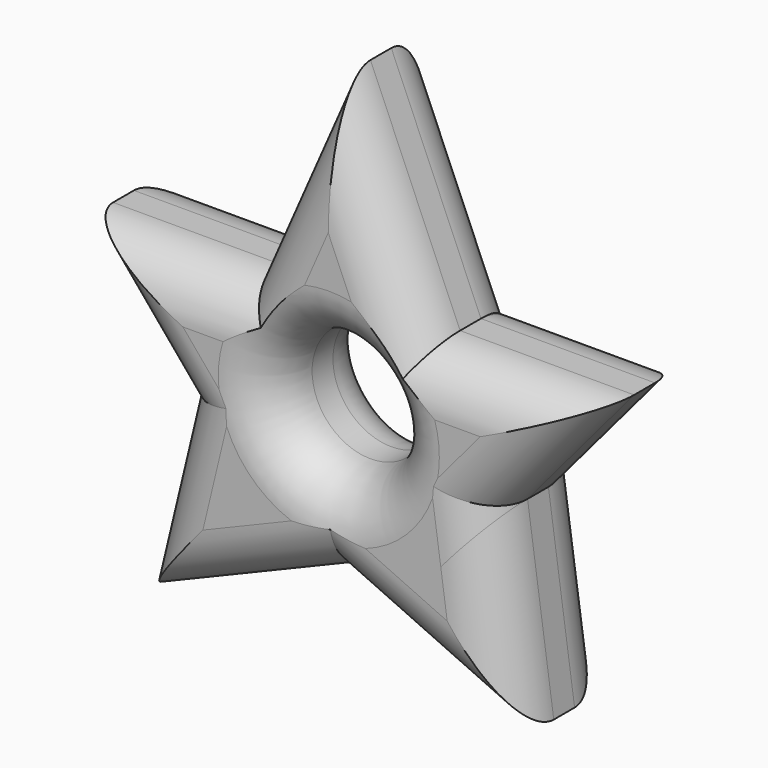
from build123d import *

# Parameters (mm, degrees)
F0_R          = 5.6926313443
F1_DEPTH      = 12.7
F2_T4_DEPTH   = 43.6889551243
F2_T9_DEPTH   = 41.5057154141
F2_T14_DEPTH  = 42.3716066055
F2_T19_DEPTH  = 47.5765515209
F2_T24_DEPTH  = 47.6597095959
F2_T29_DEPTH  = 41.5552379071
F2_T34_DEPTH  = 40.9570702629
F2_T39_DEPTH  = 44.4053400631
F2_T44_DEPTH  = 46.5690535596
F2_T49_DEPTH  = 45.0341334131
F2_T56_DEPTH  = 43.6889551243
F2_T61_DEPTH  = 41.5057154141
F2_T66_DEPTH  = 42.3716066055
F2_T71_DEPTH  = 47.5765515209
F2_T76_DEPTH  = 47.6597095959
F2_T81_DEPTH  = 41.5552379071
F2_T86_DEPTH  = 40.9570702629
F2_T91_DEPTH  = 44.4053400631
F2_T96_DEPTH  = 46.5690535596
F2_T101_DEPTH = 45.0341334131
F2_T109_DEPTH = 43.6889551243
F2_T113_DEPTH = 41.5057154141
F2_T120_DEPTH = 42.3716066055
F2_T124_DEPTH = 47.5765515209
F2_T131_DEPTH = 47.6597095959
F2_T135_DEPTH = 41.5552379071
F2_T142_DEPTH = 40.9570702629
F2_T146_DEPTH = 44.4053400631
F2_T153_DEPTH = 46.5690535596
F2_T157_DEPTH = 45.0341334131
F2_T164_DEPTH = 43.6889551243
F2_T168_DEPTH = 41.5057154141
F2_T175_DEPTH = 42.3716066055
F2_T179_DEPTH = 47.5765515209
F2_T186_DEPTH = 47.6597095959
F2_T190_DEPTH = 41.5552379071
F2_T197_DEPTH = 40.9570702629
F2_T201_DEPTH = 44.4053400631
F2_T208_DEPTH = 46.5690535596
F2_T212_DEPTH = 45.0341334131


# Not quite as in the source:
# - a fillet or chamfer that OpenCascade refuses, or shapes differently, is made with other operations: its cross-section is extruded or revolved along the edge and cut away or added


with BuildPart() as f1:
    # F0 (on Front) → F1 (new body)
    with BuildSketch(Plane.XZ):
        Polygon((25.7036406547, 22.2720243037), (8.7320340492, 22.2720243037), (0, 42.6570928276), (-8.9411214382, 22.2720243037), (-25.0963593453, 22.2720243037), (-15.1141012942, 10.3398426354), (-19.5402633399, -8.1429071724), (0, 0), (17.8659524701, -8.1429071724), (15.3123920323, 9.9669025623), align=None)
        with Locations((0, 14.1210428621)):
            Circle(F0_R, mode=Mode.SUBTRACT)
    extrude(amount=F1_DEPTH)

    # F2: fillet of radius 5.08 on 22 edges, made by hand


with BuildPart() as f2_tool2:
    # F2_s3 → F2_t4 (new body)
    with BuildSketch(Plane(origin=(3.2473042237, 0, -23.0298295556), x_dir=(0, 1, 0), z_dir=(-0.1396230906, 0, 0.9902047226))):
        with BuildLine():
            ThreePointArc((-7.62, -16.5540126433), (-11.2121024484, -15.0661150917), (-12.7, -11.4740126433))
            Line((-12.7, -11.4740126433), (-12.7, -16.5540126433))
            Line((-12.7, -16.5540126433), (-7.62, -16.5540126433))
        make_face()
    extrude(amount=F2_T4_DEPTH)

    split(bisect_by=Plane(origin=(4.0252181101, 0, -3.3991571169), x_dir=(0, 1, 0), z_dir=(0.7640220521, 0, -0.64519013)), keep=Keep.TOP)


with BuildPart() as f1_1:
    add(f1.part)

    # F2_t1: cut F2_tool2
    add(f2_tool2.part, mode=Mode.SUBTRACT)


with BuildPart() as f2_tool7:
    # F2_s8 → F2_t9 (new body)
    with BuildSketch(Plane(origin=(3.0932592707, 0, 3.6629796175), x_dir=(0, 1, 0), z_dir=(0.64519013, 0, 0.7640220521))):
        with BuildLine():
            ThreePointArc((-7.62, -5.2684580229), (-11.2121024484, -3.7805604713), (-12.7, -0.1884580229))
            Line((-12.7, -0.1884580229), (-12.7, -5.2684580229))
            Line((-12.7, -5.2684580229), (-7.62, -5.2684580229))
        make_face()
    extrude(amount=F2_T9_DEPTH)

    split(bisect_by=Plane(origin=(16.3918614967, 0, 2.3113224066), x_dir=(0, 1, 0), z_dir=(0.9902047226, 0, 0.1396230906)), keep=Keep.TOP)


with BuildPart() as f1_2:
    add(f1_1.part)

    # F2_t6: cut F2_tool7
    add(f2_tool7.part, mode=Mode.SUBTRACT)


with BuildPart() as f2_tool12:
    # F2_s13 → F2_t14 (new body)
    with BuildSketch(Plane.YZ.offset(38.4036406547)):
        with BuildLine():
            ThreePointArc((-7.62, 22.2720243037), (-11.2121024484, 20.7841267521), (-12.7, 17.1920243037))
            Line((-12.7, 17.1920243037), (-12.7, 22.2720243037))
            Line((-12.7, 22.2720243037), (-7.62, 22.2720243037))
        make_face()
    extrude(amount=-F2_T14_DEPTH)

    split(bisect_by=Plane(origin=(15.4394143514, 0, 6.6135412622), x_dir=(0, 1, 0), z_dir=(0.9192172419, 0, 0.3937507615)), keep=Keep.TOP)


with BuildPart() as f1_3:
    add(f1_2.part)

    # F2_t11: cut F2_tool12
    add(f2_tool12.part, mode=Mode.SUBTRACT)


with BuildPart() as f2_tool17:
    # F2_s18 → F2_t19 (new body)
    with BuildSketch(Plane(origin=(-1.706745631, 0, 3.9844240694), x_dir=(0, 1, 0), z_dir=(-0.3937507615, 0, 0.9192172419))):
        with BuildLine():
            ThreePointArc((-7.62, -16.7962627849), (-11.2121024484, -15.3083652333), (-12.7, -11.7162627849))
            Line((-12.7, -11.7162627849), (-12.7, -16.7962627849))
            Line((-12.7, -16.7962627849), (-7.62, -16.7962627849))
        make_face()
    extrude(amount=F2_T19_DEPTH)

    split(bisect_by=Plane.XY.offset(22.2720243037), keep=Keep.TOP)


with BuildPart() as f1_4:
    add(f1_3.part)

    # F2_t16: cut F2_tool17
    add(f2_tool17.part, mode=Mode.SUBTRACT)


with BuildPart() as f2_tool22:
    # F2_s23 → F2_t24 (new body)
    with BuildSketch(Plane(origin=(20.7924554538, 0, 47.4051976742), x_dir=(0, 1, 0), z_dir=(-0.40167287, 0, -0.9157832197))):
        with BuildLine():
            ThreePointArc((-7.62, -17.1341969008), (-11.2121024484, -15.6462993492), (-12.7, -12.0541969008))
            Line((-12.7, -12.0541969008), (-12.7, -17.1341969008))
            Line((-12.7, -17.1341969008), (-7.62, -17.1341969008))
        make_face()
    extrude(amount=F2_T24_DEPTH)

    split(bisect_by=Plane.XY.offset(22.2720243037), keep=Keep.TOP)


with BuildPart() as f1_5:
    add(f1_4.part)

    # F2_t21: cut F2_tool22
    add(f2_tool22.part, mode=Mode.SUBTRACT)


with BuildPart() as f2_tool27:
    # F2_s28 → F2_t29 (new body)
    with BuildSketch(Plane.YZ.offset(3.7588785618)):
        with BuildLine():
            ThreePointArc((-7.62, 22.2720243037), (-11.2121024484, 20.7841267521), (-12.7, 17.1920243037))
            Line((-12.7, 17.1920243037), (-12.7, 22.2720243037))
            Line((-12.7, 22.2720243037), (-7.62, 22.2720243037))
        make_face()
    extrude(amount=-F2_T29_DEPTH)

    split(bisect_by=Plane(origin=(-15.6912100052, 0, 6.8823420438), x_dir=(0, 1, 0), z_dir=(-0.9157832197, 0, 0.40167287)), keep=Keep.TOP)


with BuildPart() as f1_6:
    add(f1_5.part)

    # F2_t26: cut F2_tool27
    add(f2_tool27.part, mode=Mode.SUBTRACT)


with BuildPart() as f2_tool32:
    # F2_s33 → F2_t34 (new body)
    with BuildSketch(Plane(origin=(-29.4427441593, 0, 35.1940583308), x_dir=(0, 1, 0), z_dir=(0.6416541085, 0, -0.7669941362))):
        with BuildLine():
            ThreePointArc((-7.62, -4.9578245582), (-11.2121024484, -3.4699270066), (-12.7, 0.1221754418))
            Line((-12.7, 0.1221754418), (-12.7, -4.9578245582))
            Line((-12.7, -4.9578245582), (-7.62, -4.9578245582))
        make_face()
    extrude(amount=F2_T34_DEPTH)

    split(bisect_by=Plane(origin=(-16.6361796063, 0, 3.9839540936), x_dir=(0, 1, 0), z_dir=(-0.9725029779, 0, 0.2328904419)), keep=Keep.TOP)


with BuildPart() as f1_7:
    add(f1_6.part)

    # F2_t31: cut F2_tool32
    add(f2_tool32.part, mode=Mode.SUBTRACT)


with BuildPart() as f2_tool37:
    # F2_s38 → F2_t39 (new body)
    with BuildSketch(Plane(origin=(4.4797869241, 0, 18.7066763614), x_dir=(0, 1, 0), z_dir=(-0.2328904419, 0, -0.9725029779))):
        with BuildLine():
            ThreePointArc((-7.62, -17.1065590378), (-11.2121024484, -15.6186614862), (-12.7, -12.0265590378))
            Line((-12.7, -12.0265590378), (-12.7, -17.1065590378))
            Line((-12.7, -17.1065590378), (-7.62, -17.1065590378))
        make_face()
    extrude(amount=F2_T39_DEPTH)

    split(bisect_by=Plane(origin=(-3.8026223645, 0, -3.1812084972), x_dir=(0, 1, 0), z_dir=(-0.7669941362, 0, -0.6416541085)), keep=Keep.TOP)


with BuildPart() as f1_8:
    add(f1_7.part)

    # F2_t36: cut F2_tool37
    add(f2_tool37.part, mode=Mode.SUBTRACT)


with BuildPart() as f2_tool42:
    # F2_s43 → F2_t44 (new body)
    with BuildSketch(Plane(origin=(-31.2630993995, 0, -13.0281005893), x_dir=(0, 1, 0), z_dir=(0.9230579574, 0, 0.384660899))):
        with BuildLine():
            ThreePointArc((-7.62, 0), (-11.2121024484, 1.4878975516), (-12.7, 5.08))
            Line((-12.7, 5.08), (-12.7, 0))
            Line((-12.7, 0), (-7.62, 0))
        make_face()
    extrude(amount=F2_T44_DEPTH)

    split(bisect_by=Plane(origin=(0, 0, 0), x_dir=(0, 1, 0), z_dir=(-0.4147321912, 0, -0.90994352)), keep=Keep.TOP)


with BuildPart() as f1_9:
    add(f1_8.part)

    # F2_t41: cut F2_tool42
    add(f2_tool42.part, mode=Mode.SUBTRACT)


with BuildPart() as f2_tool47:
    # F2_s48 → F2_t49 (new body)
    with BuildSketch(Plane(origin=(-11.556282704, 0, 5.2670988281), x_dir=(0, 1, 0), z_dir=(0.90994352, 0, -0.4147321912))):
        with BuildLine():
            ThreePointArc((-7.62, 0), (-11.2121024484, 1.4878975516), (-12.7, 5.08))
            Line((-12.7, 5.08), (-12.7, 0))
            Line((-12.7, 0), (-7.62, 0))
        make_face()
    extrude(amount=F2_T49_DEPTH)

    split(bisect_by=Plane(origin=(0, 0, 0), x_dir=(0, 1, 0), z_dir=(0.384660899, 0, -0.9230579574)), keep=Keep.TOP)


with BuildPart() as f1_10:
    add(f1_9.part)

    # F2_t46: cut F2_tool47
    add(f2_tool47.part, mode=Mode.SUBTRACT)

    # F2_s51 → F2_t52 (revolve, cut)
    with BuildSketch(Plane.XY.offset(14.1210428621)):
        with BuildLine():
            ThreePointArc((5.6926313443, -7.62), (7.1805288959, -11.2121024484), (10.7726313443, -12.7))
            Line((10.7726313443, -12.7), (5.6926313443, -12.7))
            Line((5.6926313443, -12.7), (5.6926313443, -7.62))
        make_face()
    revolve(axis=Axis((0, -12.7, 14.1210428621), (0, -1, 0)), mode=Mode.SUBTRACT)


with BuildPart() as f2_tool54:
    # F2_s55 → F2_t56 (new body)
    with BuildSketch(Plane(origin=(3.2473042237, 0, -23.0298295556), x_dir=(0, 1, 0), z_dir=(-0.1396230906, 0, 0.9902047226))):
        with BuildLine():
            ThreePointArc((-5.08, -16.5540126433), (-1.4878975516, -15.0661150917), (0, -11.4740126433))
            Line((0, -11.4740126433), (0, -16.5540126433))
            Line((0, -16.5540126433), (-5.08, -16.5540126433))
        make_face()
    extrude(amount=F2_T56_DEPTH)

    split(bisect_by=Plane(origin=(4.0252181101, 0, -3.3991571169), x_dir=(0, 1, 0), z_dir=(0.7640220521, 0, -0.64519013)), keep=Keep.TOP)


with BuildPart() as f1_11:
    add(f1_10.part)

    # F2_t53: cut F2_tool54
    add(f2_tool54.part, mode=Mode.SUBTRACT)


with BuildPart() as f2_tool59:
    # F2_s60 → F2_t61 (new body)
    with BuildSketch(Plane(origin=(3.0932592707, 0, 3.6629796175), x_dir=(0, 1, 0), z_dir=(0.64519013, 0, 0.7640220521))):
        with BuildLine():
            ThreePointArc((-5.08, -5.2684580229), (-1.4878975516, -3.7805604713), (0, -0.1884580229))
            Line((0, -0.1884580229), (0, -5.2684580229))
            Line((0, -5.2684580229), (-5.08, -5.2684580229))
        make_face()
    extrude(amount=F2_T61_DEPTH)

    split(bisect_by=Plane(origin=(16.3918614967, 0, 2.3113224066), x_dir=(0, 1, 0), z_dir=(0.9902047226, 0, 0.1396230906)), keep=Keep.TOP)


with BuildPart() as f1_12:
    add(f1_11.part)

    # F2_t58: cut F2_tool59
    add(f2_tool59.part, mode=Mode.SUBTRACT)


with BuildPart() as f2_tool64:
    # F2_s65 → F2_t66 (new body)
    with BuildSketch(Plane.YZ.offset(38.4036406547)):
        with BuildLine():
            ThreePointArc((-5.08, 22.2720243037), (-1.4878975516, 20.7841267521), (0, 17.1920243037))
            Line((0, 17.1920243037), (0, 22.2720243037))
            Line((0, 22.2720243037), (-5.08, 22.2720243037))
        make_face()
    extrude(amount=-F2_T66_DEPTH)

    split(bisect_by=Plane(origin=(15.4394143514, 0, 6.6135412622), x_dir=(0, 1, 0), z_dir=(0.9192172419, 0, 0.3937507615)), keep=Keep.TOP)


with BuildPart() as f1_13:
    add(f1_12.part)

    # F2_t63: cut F2_tool64
    add(f2_tool64.part, mode=Mode.SUBTRACT)


with BuildPart() as f2_tool69:
    # F2_s70 → F2_t71 (new body)
    with BuildSketch(Plane(origin=(-1.706745631, 0, 3.9844240694), x_dir=(0, 1, 0), z_dir=(-0.3937507615, 0, 0.9192172419))):
        with BuildLine():
            ThreePointArc((-5.08, -16.7962627849), (-1.4878975516, -15.3083652333), (0, -11.7162627849))
            Line((0, -11.7162627849), (0, -16.7962627849))
            Line((0, -16.7962627849), (-5.08, -16.7962627849))
        make_face()
    extrude(amount=F2_T71_DEPTH)

    split(bisect_by=Plane.XY.offset(22.2720243037), keep=Keep.TOP)


with BuildPart() as f1_14:
    add(f1_13.part)

    # F2_t68: cut F2_tool69
    add(f2_tool69.part, mode=Mode.SUBTRACT)


with BuildPart() as f2_tool74:
    # F2_s75 → F2_t76 (new body)
    with BuildSketch(Plane(origin=(20.7924554538, 0, 47.4051976742), x_dir=(0, 1, 0), z_dir=(-0.40167287, 0, -0.9157832197))):
        with BuildLine():
            ThreePointArc((-5.08, -17.1341969008), (-1.4878975516, -15.6462993492), (0, -12.0541969008))
            Line((0, -12.0541969008), (0, -17.1341969008))
            Line((0, -17.1341969008), (-5.08, -17.1341969008))
        make_face()
    extrude(amount=F2_T76_DEPTH)

    split(bisect_by=Plane.XY.offset(22.2720243037), keep=Keep.TOP)


with BuildPart() as f1_15:
    add(f1_14.part)

    # F2_t73: cut F2_tool74
    add(f2_tool74.part, mode=Mode.SUBTRACT)


with BuildPart() as f2_tool79:
    # F2_s80 → F2_t81 (new body)
    with BuildSketch(Plane.YZ.offset(3.7588785618)):
        with BuildLine():
            ThreePointArc((-5.08, 22.2720243037), (-1.4878975516, 20.7841267521), (0, 17.1920243037))
            Line((0, 17.1920243037), (0, 22.2720243037))
            Line((0, 22.2720243037), (-5.08, 22.2720243037))
        make_face()
    extrude(amount=-F2_T81_DEPTH)

    split(bisect_by=Plane(origin=(-15.6912100052, 0, 6.8823420438), x_dir=(0, 1, 0), z_dir=(-0.9157832197, 0, 0.40167287)), keep=Keep.TOP)


with BuildPart() as f1_16:
    add(f1_15.part)

    # F2_t78: cut F2_tool79
    add(f2_tool79.part, mode=Mode.SUBTRACT)


with BuildPart() as f2_tool84:
    # F2_s85 → F2_t86 (new body)
    with BuildSketch(Plane(origin=(-29.4427441593, 0, 35.1940583308), x_dir=(0, 1, 0), z_dir=(0.6416541085, 0, -0.7669941362))):
        with BuildLine():
            ThreePointArc((-5.08, -4.9578245582), (-1.4878975516, -3.4699270066), (0, 0.1221754418))
            Line((0, 0.1221754418), (0, -4.9578245582))
            Line((0, -4.9578245582), (-5.08, -4.9578245582))
        make_face()
    extrude(amount=F2_T86_DEPTH)

    split(bisect_by=Plane(origin=(-16.6361796063, 0, 3.9839540936), x_dir=(0, 1, 0), z_dir=(-0.9725029779, 0, 0.2328904419)), keep=Keep.TOP)


with BuildPart() as f1_17:
    add(f1_16.part)

    # F2_t83: cut F2_tool84
    add(f2_tool84.part, mode=Mode.SUBTRACT)


with BuildPart() as f2_tool89:
    # F2_s90 → F2_t91 (new body)
    with BuildSketch(Plane(origin=(4.4797869241, 0, 18.7066763614), x_dir=(0, 1, 0), z_dir=(-0.2328904419, 0, -0.9725029779))):
        with BuildLine():
            ThreePointArc((-5.08, -17.1065590378), (-1.4878975516, -15.6186614862), (0, -12.0265590378))
            Line((0, -12.0265590378), (0, -17.1065590378))
            Line((0, -17.1065590378), (-5.08, -17.1065590378))
        make_face()
    extrude(amount=F2_T91_DEPTH)

    split(bisect_by=Plane(origin=(-3.8026223645, 0, -3.1812084972), x_dir=(0, 1, 0), z_dir=(-0.7669941362, 0, -0.6416541085)), keep=Keep.TOP)


with BuildPart() as f1_18:
    add(f1_17.part)

    # F2_t88: cut F2_tool89
    add(f2_tool89.part, mode=Mode.SUBTRACT)


with BuildPart() as f2_tool94:
    # F2_s95 → F2_t96 (new body)
    with BuildSketch(Plane(origin=(-31.2630993995, 0, -13.0281005893), x_dir=(0, 1, 0), z_dir=(0.9230579574, 0, 0.384660899))):
        with BuildLine():
            ThreePointArc((-5.08, 0), (-1.4878975516, 1.4878975516), (0, 5.08))
            Line((0, 5.08), (0, 0))
            Line((0, 0), (-5.08, 0))
        make_face()
    extrude(amount=F2_T96_DEPTH)

    split(bisect_by=Plane(origin=(0, 0, 0), x_dir=(0, 1, 0), z_dir=(-0.4147321912, 0, -0.90994352)), keep=Keep.TOP)


with BuildPart() as f1_19:
    add(f1_18.part)

    # F2_t93: cut F2_tool94
    add(f2_tool94.part, mode=Mode.SUBTRACT)


with BuildPart() as f2_tool99:
    # F2_s100 → F2_t101 (new body)
    with BuildSketch(Plane(origin=(-11.556282704, 0, 5.2670988281), x_dir=(0, 1, 0), z_dir=(0.90994352, 0, -0.4147321912))):
        with BuildLine():
            ThreePointArc((-5.08, 0), (-1.4878975516, 1.4878975516), (0, 5.08))
            Line((0, 5.08), (0, 0))
            Line((0, 0), (-5.08, 0))
        make_face()
    extrude(amount=F2_T101_DEPTH)

    split(bisect_by=Plane(origin=(0, 0, 0), x_dir=(0, 1, 0), z_dir=(0.384660899, 0, -0.9230579574)), keep=Keep.TOP)


with BuildPart() as f1_20:
    add(f1_19.part)

    # F2_t98: cut F2_tool99
    add(f2_tool99.part, mode=Mode.SUBTRACT)

    # F2_s103 → F2_t104 (revolve, cut)
    with BuildSketch(Plane.XY.offset(14.1210428621)):
        with BuildLine():
            ThreePointArc((5.6926313443, -5.08), (7.1805288959, -1.4878975516), (10.7726313443, 0))
            Line((10.7726313443, 0), (5.6926313443, 0))
            Line((5.6926313443, 0), (5.6926313443, -5.08))
        make_face()
    revolve(axis=Axis((0, 0, 14.1210428621), (0, -1, 0)), mode=Mode.SUBTRACT)


with BuildPart() as f2_tool107:
    # F2_s108 → F2_t109 (new body)
    with BuildSketch(Plane(origin=(3.2473042237, 0, -23.0298295556), x_dir=(0, 1, 0), z_dir=(-0.1396230906, 0, 0.9902047226))):
        with BuildLine():
            ThreePointArc((-7.62, -16.5540126433), (-11.2121024484, -15.0661150917), (-12.7, -11.4740126433))
            Line((-12.7, -11.4740126433), (-12.7, -16.5540126433))
            Line((-12.7, -16.5540126433), (-7.62, -16.5540126433))
        make_face()
    extrude(amount=F2_T109_DEPTH)

    split(bisect_by=Plane(origin=(4.0252181101, 0, -3.3991571169), x_dir=(0, 1, 0), z_dir=(-0.7640220521, 0, 0.64519013)), keep=Keep.TOP)


with BuildPart() as f2_tool111:
    # F2_s112 → F2_t113 (new body)
    with BuildSketch(Plane(origin=(3.0932592707, 0, 3.6629796175), x_dir=(0, 1, 0), z_dir=(0.64519013, 0, 0.7640220521))):
        with BuildLine():
            ThreePointArc((-7.62, -5.2684580229), (-11.2121024484, -3.7805604713), (-12.7, -0.1884580229))
            Line((-12.7, -0.1884580229), (-12.7, -5.2684580229))
            Line((-12.7, -5.2684580229), (-7.62, -5.2684580229))
        make_face()
    extrude(amount=F2_T113_DEPTH)

    split(bisect_by=Plane(origin=(16.3918614967, 0, 2.3113224066), x_dir=(0, 1, 0), z_dir=(-0.9902047226, 0, -0.1396230906)), keep=Keep.TOP)


with BuildPart() as f2_tool107_1:
    add(f2_tool107.part)

    # F2_t115: intersect F2_tool111
    add(f2_tool111.part, mode=Mode.INTERSECT)


with BuildPart() as f1_21:
    add(f1_20.part)

    # F2_t105: cut F2_tool107
    add(f2_tool107_1.part, mode=Mode.SUBTRACT)


with BuildPart() as f2_tool118:
    # F2_s119 → F2_t120 (new body)
    with BuildSketch(Plane.YZ.offset(38.4036406547)):
        with BuildLine():
            ThreePointArc((-7.62, 22.2720243037), (-11.2121024484, 20.7841267521), (-12.7, 17.1920243037))
            Line((-12.7, 17.1920243037), (-12.7, 22.2720243037))
            Line((-12.7, 22.2720243037), (-7.62, 22.2720243037))
        make_face()
    extrude(amount=-F2_T120_DEPTH)

    split(bisect_by=Plane(origin=(15.4394143514, 0, 6.6135412622), x_dir=(0, 1, 0), z_dir=(-0.9192172419, 0, -0.3937507615)), keep=Keep.TOP)


with BuildPart() as f2_tool122:
    # F2_s123 → F2_t124 (new body)
    with BuildSketch(Plane(origin=(-1.706745631, 0, 3.9844240694), x_dir=(0, 1, 0), z_dir=(-0.3937507615, 0, 0.9192172419))):
        with BuildLine():
            ThreePointArc((-7.62, -16.7962627849), (-11.2121024484, -15.3083652333), (-12.7, -11.7162627849))
            Line((-12.7, -11.7162627849), (-12.7, -16.7962627849))
            Line((-12.7, -16.7962627849), (-7.62, -16.7962627849))
        make_face()
    extrude(amount=F2_T124_DEPTH)

    split(bisect_by=Plane.XY.offset(22.2720243037), keep=Keep.BOTTOM)


with BuildPart() as f2_tool118_1:
    add(f2_tool118.part)

    # F2_t126: intersect F2_tool122
    add(f2_tool122.part, mode=Mode.INTERSECT)


with BuildPart() as f1_22:
    add(f1_21.part)

    # F2_t116: cut F2_tool118
    add(f2_tool118_1.part, mode=Mode.SUBTRACT)


with BuildPart() as f2_tool129:
    # F2_s130 → F2_t131 (new body)
    with BuildSketch(Plane(origin=(20.7924554538, 0, 47.4051976742), x_dir=(0, 1, 0), z_dir=(-0.40167287, 0, -0.9157832197))):
        with BuildLine():
            ThreePointArc((-7.62, -17.1341969008), (-11.2121024484, -15.6462993492), (-12.7, -12.0541969008))
            Line((-12.7, -12.0541969008), (-12.7, -17.1341969008))
            Line((-12.7, -17.1341969008), (-7.62, -17.1341969008))
        make_face()
    extrude(amount=F2_T131_DEPTH)

    split(bisect_by=Plane.XY.offset(22.2720243037), keep=Keep.BOTTOM)


with BuildPart() as f2_tool133:
    # F2_s134 → F2_t135 (new body)
    with BuildSketch(Plane.YZ.offset(3.7588785618)):
        with BuildLine():
            ThreePointArc((-7.62, 22.2720243037), (-11.2121024484, 20.7841267521), (-12.7, 17.1920243037))
            Line((-12.7, 17.1920243037), (-12.7, 22.2720243037))
            Line((-12.7, 22.2720243037), (-7.62, 22.2720243037))
        make_face()
    extrude(amount=-F2_T135_DEPTH)

    split(bisect_by=Plane(origin=(-15.6912100052, 0, 6.8823420438), x_dir=(0, 1, 0), z_dir=(0.9157832197, 0, -0.40167287)), keep=Keep.TOP)


with BuildPart() as f2_tool129_1:
    add(f2_tool129.part)

    # F2_t137: intersect F2_tool133
    add(f2_tool133.part, mode=Mode.INTERSECT)


with BuildPart() as f1_23:
    add(f1_22.part)

    # F2_t127: cut F2_tool129
    add(f2_tool129_1.part, mode=Mode.SUBTRACT)


with BuildPart() as f2_tool140:
    # F2_s141 → F2_t142 (new body)
    with BuildSketch(Plane(origin=(-29.4427441593, 0, 35.1940583308), x_dir=(0, 1, 0), z_dir=(0.6416541085, 0, -0.7669941362))):
        with BuildLine():
            ThreePointArc((-7.62, -4.9578245582), (-11.2121024484, -3.4699270066), (-12.7, 0.1221754418))
            Line((-12.7, 0.1221754418), (-12.7, -4.9578245582))
            Line((-12.7, -4.9578245582), (-7.62, -4.9578245582))
        make_face()
    extrude(amount=F2_T142_DEPTH)

    split(bisect_by=Plane(origin=(-16.6361796063, 0, 3.9839540936), x_dir=(0, 1, 0), z_dir=(0.9725029779, 0, -0.2328904419)), keep=Keep.TOP)


with BuildPart() as f2_tool144:
    # F2_s145 → F2_t146 (new body)
    with BuildSketch(Plane(origin=(4.4797869241, 0, 18.7066763614), x_dir=(0, 1, 0), z_dir=(-0.2328904419, 0, -0.9725029779))):
        with BuildLine():
            ThreePointArc((-7.62, -17.1065590378), (-11.2121024484, -15.6186614862), (-12.7, -12.0265590378))
            Line((-12.7, -12.0265590378), (-12.7, -17.1065590378))
            Line((-12.7, -17.1065590378), (-7.62, -17.1065590378))
        make_face()
    extrude(amount=F2_T146_DEPTH)

    split(bisect_by=Plane(origin=(-3.8026223645, 0, -3.1812084972), x_dir=(0, 1, 0), z_dir=(0.7669941362, 0, 0.6416541085)), keep=Keep.TOP)


with BuildPart() as f2_tool140_1:
    add(f2_tool140.part)

    # F2_t148: intersect F2_tool144
    add(f2_tool144.part, mode=Mode.INTERSECT)


with BuildPart() as f1_24:
    add(f1_23.part)

    # F2_t138: cut F2_tool140
    add(f2_tool140_1.part, mode=Mode.SUBTRACT)


with BuildPart() as f2_tool151:
    # F2_s152 → F2_t153 (new body)
    with BuildSketch(Plane(origin=(-31.2630993995, 0, -13.0281005893), x_dir=(0, 1, 0), z_dir=(0.9230579574, 0, 0.384660899))):
        with BuildLine():
            ThreePointArc((-7.62, 0), (-11.2121024484, 1.4878975516), (-12.7, 5.08))
            Line((-12.7, 5.08), (-12.7, 0))
            Line((-12.7, 0), (-7.62, 0))
        make_face()
    extrude(amount=F2_T153_DEPTH)

    split(bisect_by=Plane(origin=(0, 0, 0), x_dir=(0, 1, 0), z_dir=(0.4147321912, 0, 0.90994352)), keep=Keep.TOP)


with BuildPart() as f2_tool155:
    # F2_s156 → F2_t157 (new body)
    with BuildSketch(Plane(origin=(-11.556282704, 0, 5.2670988281), x_dir=(0, 1, 0), z_dir=(0.90994352, 0, -0.4147321912))):
        with BuildLine():
            ThreePointArc((-7.62, 0), (-11.2121024484, 1.4878975516), (-12.7, 5.08))
            Line((-12.7, 5.08), (-12.7, 0))
            Line((-12.7, 0), (-7.62, 0))
        make_face()
    extrude(amount=F2_T157_DEPTH)

    split(bisect_by=Plane(origin=(0, 0, 0), x_dir=(0, 1, 0), z_dir=(-0.384660899, 0, 0.9230579574)), keep=Keep.TOP)


with BuildPart() as f2_tool151_1:
    add(f2_tool151.part)

    # F2_t159: intersect F2_tool155
    add(f2_tool155.part, mode=Mode.INTERSECT)


with BuildPart() as f1_25:
    add(f1_24.part)

    # F2_t149: cut F2_tool151
    add(f2_tool151_1.part, mode=Mode.SUBTRACT)


with BuildPart() as f2_tool162:
    # F2_s163 → F2_t164 (new body)
    with BuildSketch(Plane(origin=(3.2473042237, 0, -23.0298295556), x_dir=(0, 1, 0), z_dir=(-0.1396230906, 0, 0.9902047226))):
        with BuildLine():
            ThreePointArc((-5.08, -16.5540126433), (-1.4878975516, -15.0661150917), (0, -11.4740126433))
            Line((0, -11.4740126433), (0, -16.5540126433))
            Line((0, -16.5540126433), (-5.08, -16.5540126433))
        make_face()
    extrude(amount=F2_T164_DEPTH)

    split(bisect_by=Plane(origin=(4.0252181101, 0, -3.3991571169), x_dir=(0, 1, 0), z_dir=(-0.7640220521, 0, 0.64519013)), keep=Keep.TOP)


with BuildPart() as f2_tool166:
    # F2_s167 → F2_t168 (new body)
    with BuildSketch(Plane(origin=(3.0932592707, 0, 3.6629796175), x_dir=(0, 1, 0), z_dir=(0.64519013, 0, 0.7640220521))):
        with BuildLine():
            ThreePointArc((-5.08, -5.2684580229), (-1.4878975516, -3.7805604713), (0, -0.1884580229))
            Line((0, -0.1884580229), (0, -5.2684580229))
            Line((0, -5.2684580229), (-5.08, -5.2684580229))
        make_face()
    extrude(amount=F2_T168_DEPTH)

    split(bisect_by=Plane(origin=(16.3918614967, 0, 2.3113224066), x_dir=(0, 1, 0), z_dir=(-0.9902047226, 0, -0.1396230906)), keep=Keep.TOP)


with BuildPart() as f2_tool162_1:
    add(f2_tool162.part)

    # F2_t170: intersect F2_tool166
    add(f2_tool166.part, mode=Mode.INTERSECT)


with BuildPart() as f1_26:
    add(f1_25.part)

    # F2_t160: cut F2_tool162
    add(f2_tool162_1.part, mode=Mode.SUBTRACT)


with BuildPart() as f2_tool173:
    # F2_s174 → F2_t175 (new body)
    with BuildSketch(Plane.YZ.offset(38.4036406547)):
        with BuildLine():
            ThreePointArc((-5.08, 22.2720243037), (-1.4878975516, 20.7841267521), (0, 17.1920243037))
            Line((0, 17.1920243037), (0, 22.2720243037))
            Line((0, 22.2720243037), (-5.08, 22.2720243037))
        make_face()
    extrude(amount=-F2_T175_DEPTH)

    split(bisect_by=Plane(origin=(15.4394143514, 0, 6.6135412622), x_dir=(0, 1, 0), z_dir=(-0.9192172419, 0, -0.3937507615)), keep=Keep.TOP)


with BuildPart() as f2_tool177:
    # F2_s178 → F2_t179 (new body)
    with BuildSketch(Plane(origin=(-1.706745631, 0, 3.9844240694), x_dir=(0, 1, 0), z_dir=(-0.3937507615, 0, 0.9192172419))):
        with BuildLine():
            ThreePointArc((-5.08, -16.7962627849), (-1.4878975516, -15.3083652333), (0, -11.7162627849))
            Line((0, -11.7162627849), (0, -16.7962627849))
            Line((0, -16.7962627849), (-5.08, -16.7962627849))
        make_face()
    extrude(amount=F2_T179_DEPTH)

    split(bisect_by=Plane.XY.offset(22.2720243037), keep=Keep.BOTTOM)


with BuildPart() as f2_tool173_1:
    add(f2_tool173.part)

    # F2_t181: intersect F2_tool177
    add(f2_tool177.part, mode=Mode.INTERSECT)


with BuildPart() as f1_27:
    add(f1_26.part)

    # F2_t171: cut F2_tool173
    add(f2_tool173_1.part, mode=Mode.SUBTRACT)


with BuildPart() as f2_tool184:
    # F2_s185 → F2_t186 (new body)
    with BuildSketch(Plane(origin=(20.7924554538, 0, 47.4051976742), x_dir=(0, 1, 0), z_dir=(-0.40167287, 0, -0.9157832197))):
        with BuildLine():
            ThreePointArc((-5.08, -17.1341969008), (-1.4878975516, -15.6462993492), (0, -12.0541969008))
            Line((0, -12.0541969008), (0, -17.1341969008))
            Line((0, -17.1341969008), (-5.08, -17.1341969008))
        make_face()
    extrude(amount=F2_T186_DEPTH)

    split(bisect_by=Plane.XY.offset(22.2720243037), keep=Keep.BOTTOM)


with BuildPart() as f2_tool188:
    # F2_s189 → F2_t190 (new body)
    with BuildSketch(Plane.YZ.offset(3.7588785618)):
        with BuildLine():
            ThreePointArc((-5.08, 22.2720243037), (-1.4878975516, 20.7841267521), (0, 17.1920243037))
            Line((0, 17.1920243037), (0, 22.2720243037))
            Line((0, 22.2720243037), (-5.08, 22.2720243037))
        make_face()
    extrude(amount=-F2_T190_DEPTH)

    split(bisect_by=Plane(origin=(-15.6912100052, 0, 6.8823420438), x_dir=(0, 1, 0), z_dir=(0.9157832197, 0, -0.40167287)), keep=Keep.TOP)


with BuildPart() as f2_tool184_1:
    add(f2_tool184.part)

    # F2_t192: intersect F2_tool188
    add(f2_tool188.part, mode=Mode.INTERSECT)


with BuildPart() as f1_28:
    add(f1_27.part)

    # F2_t182: cut F2_tool184
    add(f2_tool184_1.part, mode=Mode.SUBTRACT)


with BuildPart() as f2_tool195:
    # F2_s196 → F2_t197 (new body)
    with BuildSketch(Plane(origin=(-29.4427441593, 0, 35.1940583308), x_dir=(0, 1, 0), z_dir=(0.6416541085, 0, -0.7669941362))):
        with BuildLine():
            ThreePointArc((-5.08, -4.9578245582), (-1.4878975516, -3.4699270066), (0, 0.1221754418))
            Line((0, 0.1221754418), (0, -4.9578245582))
            Line((0, -4.9578245582), (-5.08, -4.9578245582))
        make_face()
    extrude(amount=F2_T197_DEPTH)

    split(bisect_by=Plane(origin=(-16.6361796063, 0, 3.9839540936), x_dir=(0, 1, 0), z_dir=(0.9725029779, 0, -0.2328904419)), keep=Keep.TOP)


with BuildPart() as f2_tool199:
    # F2_s200 → F2_t201 (new body)
    with BuildSketch(Plane(origin=(4.4797869241, 0, 18.7066763614), x_dir=(0, 1, 0), z_dir=(-0.2328904419, 0, -0.9725029779))):
        with BuildLine():
            ThreePointArc((-5.08, -17.1065590378), (-1.4878975516, -15.6186614862), (0, -12.0265590378))
            Line((0, -12.0265590378), (0, -17.1065590378))
            Line((0, -17.1065590378), (-5.08, -17.1065590378))
        make_face()
    extrude(amount=F2_T201_DEPTH)

    split(bisect_by=Plane(origin=(-3.8026223645, 0, -3.1812084972), x_dir=(0, 1, 0), z_dir=(0.7669941362, 0, 0.6416541085)), keep=Keep.TOP)


with BuildPart() as f2_tool195_1:
    add(f2_tool195.part)

    # F2_t203: intersect F2_tool199
    add(f2_tool199.part, mode=Mode.INTERSECT)


with BuildPart() as f1_29:
    add(f1_28.part)

    # F2_t193: cut F2_tool195
    add(f2_tool195_1.part, mode=Mode.SUBTRACT)


with BuildPart() as f2_tool206:
    # F2_s207 → F2_t208 (new body)
    with BuildSketch(Plane(origin=(-31.2630993995, 0, -13.0281005893), x_dir=(0, 1, 0), z_dir=(0.9230579574, 0, 0.384660899))):
        with BuildLine():
            ThreePointArc((-5.08, 0), (-1.4878975516, 1.4878975516), (0, 5.08))
            Line((0, 5.08), (0, 0))
            Line((0, 0), (-5.08, 0))
        make_face()
    extrude(amount=F2_T208_DEPTH)

    split(bisect_by=Plane(origin=(0, 0, 0), x_dir=(0, 1, 0), z_dir=(0.4147321912, 0, 0.90994352)), keep=Keep.TOP)


with BuildPart() as f2_tool210:
    # F2_s211 → F2_t212 (new body)
    with BuildSketch(Plane(origin=(-11.556282704, 0, 5.2670988281), x_dir=(0, 1, 0), z_dir=(0.90994352, 0, -0.4147321912))):
        with BuildLine():
            ThreePointArc((-5.08, 0), (-1.4878975516, 1.4878975516), (0, 5.08))
            Line((0, 5.08), (0, 0))
            Line((0, 0), (-5.08, 0))
        make_face()
    extrude(amount=F2_T212_DEPTH)

    split(bisect_by=Plane(origin=(0, 0, 0), x_dir=(0, 1, 0), z_dir=(-0.384660899, 0, 0.9230579574)), keep=Keep.TOP)


with BuildPart() as f2_tool206_1:
    add(f2_tool206.part)

    # F2_t214: intersect F2_tool210
    add(f2_tool210.part, mode=Mode.INTERSECT)


with BuildPart() as f1_30:
    add(f1_29.part)

    # F2_t204: cut F2_tool206
    add(f2_tool206_1.part, mode=Mode.SUBTRACT)


solid = f1_30.part
